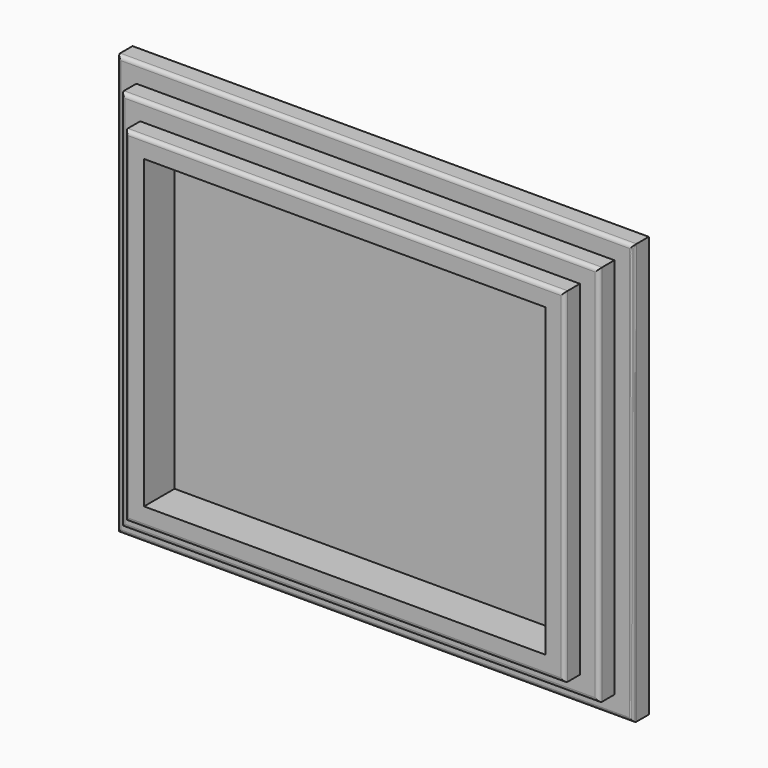
from build123d import *

# Parameters (mm, degrees)
F0_W      = 342.9
F0_H      = 279.4
F1_DEPTH  = 12.7
F2_W      = 317.5
F2_H      = 254
F3_DEPTH  = 12.7
F4_W      = 292.1
F4_H      = 228.6
F5_DEPTH  = 12.7
F6_T      = -12.7
F7_W      = 279.4
F7_H      = 3.175
F8_DEPTH  = 25.4
F9_R      = 2.54
F10_W     = 12.7
F10_H     = 12.7
F11_DEPTH = 12.7
F14_W     = 6.35
F14_H     = 12.7
F15_DEPTH = 12.7
F17_W     = 6.35
F17_H     = 12.7
F18_DEPTH = 12.7


# Not quite as in the source:
# - a feature of the source that left no trace in its solid (it failed there, or was rolled back) is left out
# - a shell that OpenCascade refuses in one call is made with other operations: the cavity is built on its own and cut out


with BuildPart() as f1:
    # F0 (on Front) → F1 (new body)
    with BuildSketch(Plane.XZ):
        Rectangle(F0_W, F0_H)
    extrude(amount=F1_DEPTH)

    # F2 (on face) → F3 (join)
    with BuildSketch(Plane.XZ.offset(12.7)):
        Rectangle(F2_W, F2_H)
    extrude(amount=F3_DEPTH)

    # F4 (on face) → F5 (join)
    with BuildSketch(Plane.XZ.offset(25.4)):
        Rectangle(F4_W, F4_H)
    extrude(amount=F5_DEPTH)

    # F6: a shell. OpenCascade refuses it in one call, so the cavity is built on its own and cut out:
    # the body offset inwards by the wall thickness, plus a prism from it out through each open face.
    f6_core = offset(f1.part, amount=F6_T, kind=Kind.INTERSECTION, mode=Mode.PRIVATE)
    f6_exits = [f6_core.faces().sort_by_distance(p)[0] for p in [
        (0, -25.4, 0),
    ]]
    add(f6_core, mode=Mode.SUBTRACT)
    extrude(f6_exits, amount=-F6_T, mode=Mode.SUBTRACT)

    # F7 (on face) → F8 (cut)
    with BuildSketch(Plane.XY.offset(127)):
        with Locations((0.0025813838, -20.3239014355)):
            Rectangle(F7_W, F7_H)
    extrude(amount=-F8_DEPTH, mode=Mode.SUBTRACT)

    # F9
    f9_edges = [f1.edges().sort_by_distance(p)[0] for p in [
        (0, -38.1, 114.3),
        (146.05, -38.1, 0),
        (158.75, -25.4, 0),
        (0, -25.4, 127),
        (0, -12.7, 139.7),
        (171.45, -12.7, 0),
        (0, -38.1, -114.3),
        (0, -25.4, -127),
        (0, -12.7, -139.7),
        (-171.45, -12.7, 0),
        (-158.75, -25.4, 0),
        (-146.05, -38.1, 0),
    ]]
    fillet(f9_edges, radius=F9_R)

    # F10 (on face) → F11 (join)
    with BuildSketch(Plane(origin=(0, 0, 0), x_dir=(-1, 0, 0), z_dir=(0, 1, 0))):
        with Locations((-139.7, 107.95)):
            Rectangle(F10_W, F10_H)
    extrude(amount=F11_DEPTH)

    # F12: F1 across plane


with BuildPart() as f1_1:
    add(f1.part)
    add(f1.part.mirror(Plane.YZ))

    # F13: F1 across plane


with BuildPart() as f1_2:
    add(f1_1.part)
    add(f1_1.part.mirror(Plane.XY))

    # F17 (on face) → F18 (join)
    with BuildSketch(Plane.YZ.offset(146.05)):
        with Locations((9.525, -120.65)):
            Rectangle(F17_W, F17_H)
    extrude(amount=-F18_DEPTH)


with BuildPart() as f15:
    # F14 (on face) → F15 (new body)
    with BuildSketch(Plane.YZ.offset(146.05)):
        with Locations((9.525, 95.25)):
            Rectangle(F14_W, F14_H)
    extrude(amount=-F15_DEPTH)


with BuildPart() as f16_1:
    # F16: instance of F15
    add(f15.part.mirror(Plane.YZ))


with BuildPart() as f19_1:
    # F19: instance of F1
    add(f1_2.part.mirror(Plane.YZ))


solid = Compound([f1_2.part, f15.part, f16_1.part, f19_1.part])
